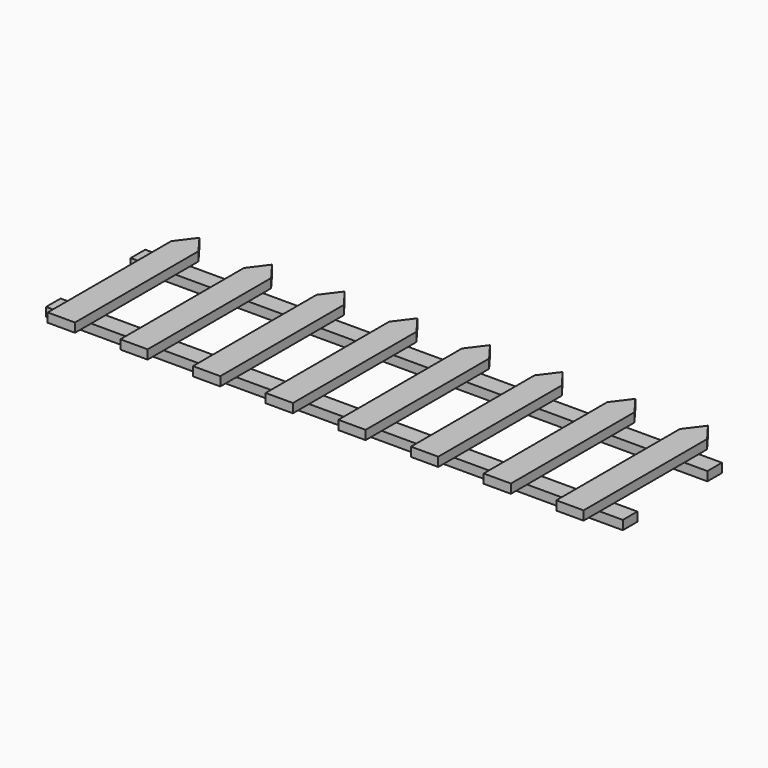
from build123d import *

# Parameters (mm, degrees)
F1_START    = 1
F0_W        = 3
F0_H        = 19
F1_DEPTH    = 1
F2_W        = 63.5
F2_H        = 2
F3_DEPTH    = 1
F4_SIZE2    = 1.5
F4_SIZE     = 2
F4_2_SIZE2  = 1.49999
F4_2_SIZE   = 1.99999
F4_3_SIZE2  = 1.5
F4_3_SIZE   = 2
F4_4_SIZE2  = 1.49999
F4_4_SIZE   = 1.99999
F4_5_SIZE2  = 1.5
F4_5_SIZE   = 2
F4_6_SIZE2  = 1.49999
F4_6_SIZE   = 1.99999
F4_7_SIZE2  = 1.5
F4_7_SIZE   = 2
F4_8_SIZE2  = 1.49999
F4_8_SIZE   = 1.99999
F4_9_SIZE2  = 1.5
F4_9_SIZE   = 2
F4_10_SIZE2 = 1.49999
F4_10_SIZE  = 1.99999
F4_11_SIZE2 = 1.5
F4_11_SIZE  = 2
F4_12_SIZE2 = 1.49999
F4_12_SIZE  = 1.99999
F4_13_SIZE2 = 1.5
F4_13_SIZE  = 2
F4_14_SIZE2 = 1.49999
F4_14_SIZE  = 1.99999
F4_15_SIZE2 = 1.5
F4_15_SIZE  = 2
F4_16_SIZE2 = 1.49999
F4_16_SIZE  = 1.99999


# Not quite as in the source:
# - a fillet or chamfer is up to 0.001 mm smaller than in the source, because OpenCascade refuses the exact size


with BuildPart() as f1:
    # F0 (on Top) → F1 (new body)
    with BuildSketch(Plane.XY.offset(F1_START)):
        with Locations((-62.5430910557, 9.5)):
            Rectangle(F0_W, F0_H)
    extrude(amount=F1_DEPTH)

    # F4
    f4_edges = [f1.edges().sort_by_distance(p)[0] for p in [
        (-64.043091, 19, 1.5),
    ]]
    f4_side = f1.faces().sort_by_distance((-64.043091, 9.5, 1.5))[0]
    chamfer(f4_edges, length=F4_SIZE, length2=F4_SIZE2, reference=f4_side)

    # F4#2 (size 2 and 1.5 in the source; OpenCascade refuses exactly that, so slightly less here)
    f4_2_edges = [f1.edges().sort_by_distance(p)[0] for p in [
        (-61.043091, 19, 1.5),
    ]]
    f4_2_side = f1.faces().sort_by_distance((-61.043091, 9.5, 1.5))[0]
    chamfer(f4_2_edges, length=F4_2_SIZE, length2=F4_2_SIZE2, reference=f4_2_side)


with BuildPart() as f1b:
    # F0 (on Top) → F1, piece 2 (new body)
    with BuildSketch(Plane.XY.offset(F1_START)):
        with Locations((-54.5430910557, 9.5)):
            Rectangle(F0_W, F0_H)
    extrude(amount=F1_DEPTH)

    # F4#3
    f4_3_edges = [f1b.edges().sort_by_distance(p)[0] for p in [
        (-56.043091, 19, 1.5),
    ]]
    f4_3_side = f1b.faces().sort_by_distance((-56.043091, 9.5, 1.5))[0]
    chamfer(f4_3_edges, length=F4_3_SIZE, length2=F4_3_SIZE2, reference=f4_3_side)

    # F4#4 (size 2 and 1.5 in the source; OpenCascade refuses exactly that, so slightly less here)
    f4_4_edges = [f1b.edges().sort_by_distance(p)[0] for p in [
        (-53.043091, 19, 1.5),
    ]]
    f4_4_side = f1b.faces().sort_by_distance((-53.043091, 9.5, 1.5))[0]
    chamfer(f4_4_edges, length=F4_4_SIZE, length2=F4_4_SIZE2, reference=f4_4_side)


with BuildPart() as f1c:
    # F0 (on Top) → F1, piece 3 (new body)
    with BuildSketch(Plane.XY.offset(F1_START)):
        with Locations((-46.5430910557, 9.5)):
            Rectangle(F0_W, F0_H)
    extrude(amount=F1_DEPTH)

    # F4#5
    f4_5_edges = [f1c.edges().sort_by_distance(p)[0] for p in [
        (-48.043091, 19, 1.5),
    ]]
    f4_5_side = f1c.faces().sort_by_distance((-48.043091, 9.5, 1.5))[0]
    chamfer(f4_5_edges, length=F4_5_SIZE, length2=F4_5_SIZE2, reference=f4_5_side)

    # F4#6 (size 2 and 1.5 in the source; OpenCascade refuses exactly that, so slightly less here)
    f4_6_edges = [f1c.edges().sort_by_distance(p)[0] for p in [
        (-45.043091, 19, 1.5),
    ]]
    f4_6_side = f1c.faces().sort_by_distance((-45.043091, 9.5, 1.5))[0]
    chamfer(f4_6_edges, length=F4_6_SIZE, length2=F4_6_SIZE2, reference=f4_6_side)


with BuildPart() as f1d:
    # F0 (on Top) → F1, piece 4 (new body)
    with BuildSketch(Plane.XY.offset(F1_START)):
        with Locations((-38.5430910557, 9.5)):
            Rectangle(F0_W, F0_H)
    extrude(amount=F1_DEPTH)

    # F4#7
    f4_7_edges = [f1d.edges().sort_by_distance(p)[0] for p in [
        (-40.043091, 19, 1.5),
    ]]
    f4_7_side = f1d.faces().sort_by_distance((-40.043091, 9.5, 1.5))[0]
    chamfer(f4_7_edges, length=F4_7_SIZE, length2=F4_7_SIZE2, reference=f4_7_side)

    # F4#8 (size 2 and 1.5 in the source; OpenCascade refuses exactly that, so slightly less here)
    f4_8_edges = [f1d.edges().sort_by_distance(p)[0] for p in [
        (-37.043091, 19, 1.5),
    ]]
    f4_8_side = f1d.faces().sort_by_distance((-37.043091, 9.5, 1.5))[0]
    chamfer(f4_8_edges, length=F4_8_SIZE, length2=F4_8_SIZE2, reference=f4_8_side)


with BuildPart() as f1e:
    # F0 (on Top) → F1, piece 5 (new body)
    with BuildSketch(Plane.XY.offset(F1_START)):
        with Locations((-30.5430910557, 9.5)):
            Rectangle(F0_W, F0_H)
    extrude(amount=F1_DEPTH)

    # F4#9
    f4_9_edges = [f1e.edges().sort_by_distance(p)[0] for p in [
        (-32.043091, 19, 1.5),
    ]]
    f4_9_side = f1e.faces().sort_by_distance((-32.043091, 9.5, 1.5))[0]
    chamfer(f4_9_edges, length=F4_9_SIZE, length2=F4_9_SIZE2, reference=f4_9_side)

    # F4#10 (size 2 and 1.5 in the source; OpenCascade refuses exactly that, so slightly less here)
    f4_10_edges = [f1e.edges().sort_by_distance(p)[0] for p in [
        (-29.043091, 19, 1.5),
    ]]
    f4_10_side = f1e.faces().sort_by_distance((-29.043091, 9.5, 1.5))[0]
    chamfer(f4_10_edges, length=F4_10_SIZE, length2=F4_10_SIZE2, reference=f4_10_side)


with BuildPart() as f1f:
    # F0 (on Top) → F1, piece 6 (new body)
    with BuildSketch(Plane.XY.offset(F1_START)):
        with Locations((-22.5430910557, 9.5)):
            Rectangle(F0_W, F0_H)
    extrude(amount=F1_DEPTH)

    # F4#15
    f4_15_edges = [f1f.edges().sort_by_distance(p)[0] for p in [
        (-24.043091, 19, 1.5),
    ]]
    f4_15_side = f1f.faces().sort_by_distance((-24.043091, 9.5, 1.5))[0]
    chamfer(f4_15_edges, length=F4_15_SIZE, length2=F4_15_SIZE2, reference=f4_15_side)

    # F4#16 (size 2 and 1.5 in the source; OpenCascade refuses exactly that, so slightly less here)
    f4_16_edges = [f1f.edges().sort_by_distance(p)[0] for p in [
        (-21.043091, 19, 1.5),
    ]]
    f4_16_side = f1f.faces().sort_by_distance((-21.043091, 9.5, 1.5))[0]
    chamfer(f4_16_edges, length=F4_16_SIZE, length2=F4_16_SIZE2, reference=f4_16_side)


with BuildPart() as f1g:
    # F0 (on Top) → F1, piece 7 (new body)
    with BuildSketch(Plane.XY.offset(F1_START)):
        with Locations((-14.5430910557, 9.5)):
            Rectangle(F0_W, F0_H)
    extrude(amount=F1_DEPTH)

    # F4#11
    f4_11_edges = [f1g.edges().sort_by_distance(p)[0] for p in [
        (-16.043091, 19, 1.5),
    ]]
    f4_11_side = f1g.faces().sort_by_distance((-16.043091, 9.5, 1.5))[0]
    chamfer(f4_11_edges, length=F4_11_SIZE, length2=F4_11_SIZE2, reference=f4_11_side)

    # F4#12 (size 2 and 1.5 in the source; OpenCascade refuses exactly that, so slightly less here)
    f4_12_edges = [f1g.edges().sort_by_distance(p)[0] for p in [
        (-13.043091, 19, 1.5),
    ]]
    f4_12_side = f1g.faces().sort_by_distance((-13.043091, 9.5, 1.5))[0]
    chamfer(f4_12_edges, length=F4_12_SIZE, length2=F4_12_SIZE2, reference=f4_12_side)


with BuildPart() as f1h:
    # F0 (on Top) → F1, piece 8 (new body)
    with BuildSketch(Plane.XY.offset(F1_START)):
        with Locations((-6.5430910557, 9.5)):
            Rectangle(F0_W, F0_H)
    extrude(amount=F1_DEPTH)

    # F4#13
    f4_13_edges = [f1h.edges().sort_by_distance(p)[0] for p in [
        (-8.043091, 19, 1.5),
    ]]
    f4_13_side = f1h.faces().sort_by_distance((-8.043091, 9.5, 1.5))[0]
    chamfer(f4_13_edges, length=F4_13_SIZE, length2=F4_13_SIZE2, reference=f4_13_side)

    # F4#14 (size 2 and 1.5 in the source; OpenCascade refuses exactly that, so slightly less here)
    f4_14_edges = [f1h.edges().sort_by_distance(p)[0] for p in [
        (-5.043091, 19, 1.5),
    ]]
    f4_14_side = f1h.faces().sort_by_distance((-5.043091, 9.5, 1.5))[0]
    chamfer(f4_14_edges, length=F4_14_SIZE, length2=F4_14_SIZE2, reference=f4_14_side)


with BuildPart() as f3:
    # F2 (on Top) → F3 (new body)
    with BuildSketch(Plane.XY):
        with Locations((-34.25, 14.8639390082)):
            Rectangle(F2_W, F2_H)
    extrude(amount=F3_DEPTH)


with BuildPart() as f3b:
    # F2 (on Top) → F3, piece 2 (new body)
    with BuildSketch(Plane.XY):
        with Locations((-34.25, 3.2210190073)):
            Rectangle(F2_W, F2_H)
    extrude(amount=F3_DEPTH)


solid = Compound([f1.part, f1b.part, f1c.part, f1d.part, f1e.part, f1f.part, f1g.part, f1h.part, f3.part, f3b.part])
